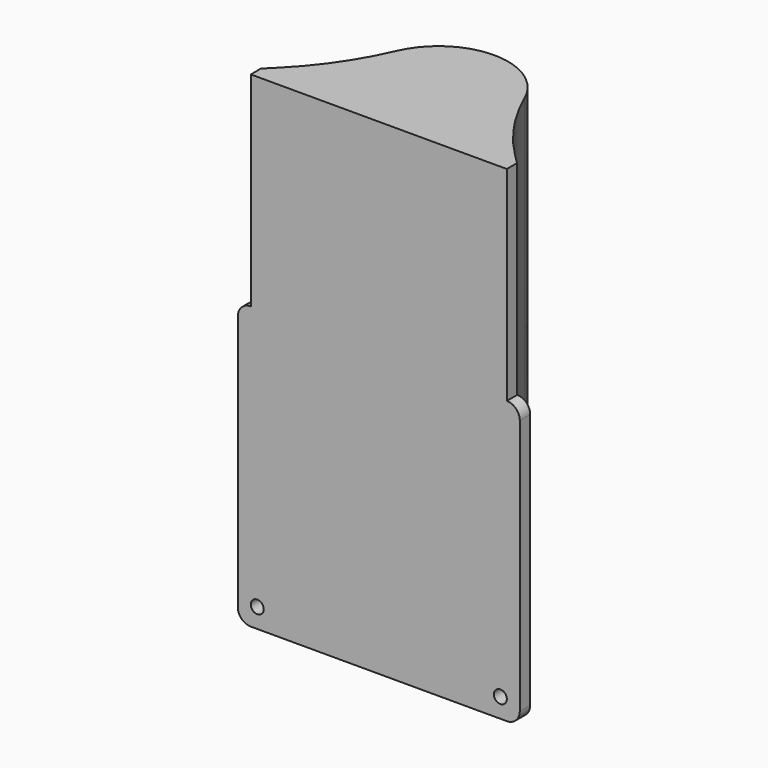
from build123d import *
from build123d import SkipClean  # not in build123d's __all__

# Parameters (mm, degrees)
F0_W           = 87
F0_H           = 87
F0_R           = 2
F1_DEPTH       = 4
F2_R           = 4
F5_DEPTH       = 43.5
F6_T1_DEPTH    = 87
F7_R           = 20.025
F8_DEPTH       = 87.001
F9_R           = 2
F10_DEPTH      = 40.501
F11_R          = 20
F12_DEPTH      = 10
F15_DEPTH      = 106.5
F15_DEPTH_BACK = 25.4
F16_R          = 20
F17_DEPTH      = 150.0010001
F18_R          = 20
F19_DEPTH      = 15


# Not quite as in the source:
# - a fillet or chamfer that OpenCascade refuses, or shapes differently, is made with other operations: its cross-section is extruded or revolved along the edge and cut away or added
# - after a boolean that leaves OpenCascade's solid faulty, fix() repairs it


with BuildPart() as f1:
    # F0 (on Front) → F1 (new body)
    with BuildSketch(Plane.XZ):
        Rectangle(F0_W, F0_H)
        with Locations((-37.5, -37.5)):
            Circle(F0_R, mode=Mode.SUBTRACT)
        with Locations((37.5, -37.5)):
            Circle(F0_R, mode=Mode.SUBTRACT)
        with Locations((-37.5, 37.5)):
            Circle(F0_R, mode=Mode.SUBTRACT)
        with Locations((37.5, 37.5)):
            Circle(F0_R, mode=Mode.SUBTRACT)
    extrude(amount=F1_DEPTH)

    # F2
    f2_edges = [f1.edges().sort_by_distance(p)[0] for p in [
        (43.5, -2, 43.5),
        (-43.5, -2, 43.5),
        (43.5, -2, -43.5),
        (-43.5, -2, -43.5),
    ]]
    fillet(f2_edges, radius=F2_R)

    # F4 (on Top) → F5 (join, symmetric)
    with BuildSketch(Plane.XY):
        with BuildLine():
            ThreePointArc((-10.0623058987, 0), (-17.7800410903, 6.9119836686), (-21.3690774705, 16.6309225295))
            Line((-21.3690774705, 16.6309225295), (-38, 0))
            Line((-38, 0), (-10.0623058987, 0))
        make_face()
        with BuildLine():
            Line((-38, 0), (-21.3690774705, 16.6309225295))
            ThreePointArc((-21.3690774705, 16.6309225295), (-21.4314768317, 17.2848321331), (-21.4738707868, 17.9403427756))
            Line((-21.4738707868, 17.9403427756), (-39.4142135624, 0))
            Line((-39.4142135624, 0), (-38, 0))
        make_face()
        with BuildLine():
            ThreePointArc((-21.4738707868, 17.9403427756), (-21.4314768317, 17.2848321331), (-21.3690774705, 16.6309225295))
            ThreePointArc((-21.3690774705, 16.6309225295), (-17.7800410903, 6.9119836686), (-10.0623058987, 0))
            Line((-10.0623058987, 0), (10.0623058987, 0))
            ThreePointArc((10.0623058987, 0), (17.7800410903, 6.9119836686), (21.3690774705, 16.6309225295))
            ThreePointArc((21.3690774705, 16.6309225295), (21.4314768317, 17.2848321331), (21.4738707868, 17.9403427756))
            Line((21.4738707868, 17.9403427756), (19.9956189847, 19.4185945777))
            ThreePointArc((19.9956189847, 19.4185945777), (13.9933575036, 33.2893647786), (0, 39))
            ThreePointArc((0, 39), (-13.9933575036, 33.2893647786), (-19.9956189847, 19.4185945777))
            Line((-19.9956189847, 19.4185945777), (-21.4738707868, 17.9403427756))
        make_face()
        with BuildLine():
            ThreePointArc((21.5, 19), (-0.5299896624, 40.493466704), (-21.4738707868, 17.9403427756))
            Line((-21.4738707868, 17.9403427756), (-19.9956189847, 19.4185945777))
            ThreePointArc((-19.9956189847, 19.4185945777), (-13.9933575036, 33.2893647786), (0, 39))
            ThreePointArc((0, 39), (13.9933575036, 33.2893647786), (19.9956189847, 19.4185945777))
            Line((19.9956189847, 19.4185945777), (21.4738707868, 17.9403427756))
            ThreePointArc((21.4738707868, 17.9403427756), (21.493466704, 18.4700103376), (21.5, 19))
        make_face()
        with BuildLine():
            Line((10.0623058987, 0), (-10.0623058987, 0))
            ThreePointArc((-10.0623058987, 0), (0, -2.5), (10.0623058987, 0))
        make_face()
        with BuildLine():
            ThreePointArc((21.3690774705, 16.6309225295), (17.7800410903, 6.9119836686), (10.0623058987, 0))
            Line((10.0623058987, 0), (38, 0))
            Line((38, 0), (21.3690774705, 16.6309225295))
        make_face()
        with BuildLine():
            Line((39.4142135624, 0), (21.4738707868, 17.9403427756))
            ThreePointArc((21.4738707868, 17.9403427756), (21.4314768317, 17.2848321331), (21.3690774705, 16.6309225295))
            Line((21.3690774705, 16.6309225295), (38, 0))
            Line((38, 0), (39.4142135624, 0))
        make_face()
    extrude(amount=F5_DEPTH, both=True)

    # F6: fillet of radius 80 on 2 edges, made by hand

    # F6_s2 → F6_t1 (join)
    with BuildSketch(Plane.XY.offset(-43.5)):
        with BuildLine():
            ThreePointArc((-36.5156161223, 2.89859744), (-26.9555540815, 14.444838104), (-19.7173340913, 27.5718572276))
            ThreePointArc((-19.7173340913, 27.5718572276), (-21.1511313524, 22.857413967), (-21.4738707868, 17.9403427756))
            Line((-21.4738707868, 17.9403427756), (-36.5156161223, 2.89859744))
        make_face()
        with BuildLine():
            ThreePointArc((19.7173340913, 27.5718572276), (26.9555540815, 14.444838104), (36.5156161223, 2.89859744))
            Line((36.5156161223, 2.89859744), (21.4738707868, 17.9403427756))
            ThreePointArc((21.4738707868, 17.9403427756), (21.1511313524, 22.857413967), (19.7173340913, 27.5718572276))
        make_face()
    extrude(amount=F6_T1_DEPTH)

    # F7 (on face) → F8 (cut, through all)
    with BuildSketch(Plane.XY.offset(43.5)):
        with Locations((0, 19)):
            Circle(F7_R)
    extrude(amount=-F8_DEPTH, mode=Mode.SUBTRACT)

    # F9 (on Front) → F10 (cut, through all)
    with BuildSketch(Plane.XZ):
        with BuildLine():
            Line((-37.5, 35.5), (-37.5, 37.5))
            Line((-37.5, 37.5), (-35.5, 37.5))
            ThreePointArc((-35.5, 37.5), (-38.9142135624, 38.9142135624), (-37.5, 35.5))
        make_face()
        with BuildLine():
            Line((-35.5, 37.5), (-37.5, 37.5))
            Line((-37.5, 37.5), (-37.5, 35.5))
            ThreePointArc((-37.5, 35.5), (-36.0857864376, 36.0857864376), (-35.5, 37.5))
        make_face()
        with BuildLine():
            ThreePointArc((39.5, 37.5), (37.5, 39.5), (35.5, 37.5))
            ThreePointArc((35.5, 37.5), (37.5, 35.5), (39.5, 37.5))
        make_face()
        with BuildLine():
            ThreePointArc((-35.5, -37.5), (-36.0857864376, -36.0857864376), (-37.5, -35.5))
            ThreePointArc((-37.5, -35.5), (-38.9142135624, -38.9142135624), (-35.5, -37.5))
        make_face()
        with Locations((37.5, -37.5)):
            Circle(F9_R)
    with SkipClean():  # cleaning this boolean's faces spoils the solid; the shape is the same uncleaned
        extrude(amount=-F10_DEPTH, mode=Mode.SUBTRACT)

    # F14 (on Top) → F15 (join, two sides)
    with BuildSketch(Plane.XY) as f15_sk:
        with BuildLine():
            Line((-39.5, -4), (39.5, -4))
            Line((39.5, -4), (39.5, 0))
            Line((39.5, 0), (39.4142135624, 0))
            Line((39.4142135624, 0), (36.5156161223, 2.89859744))
            ThreePointArc((36.5156161223, 2.89859744), (26.9555540815, 14.444838104), (19.7173340913, 27.5718572276))
            ThreePointArc((19.7173340913, 27.5718572276), (0, 40.5), (-19.7173340913, 27.5718572276))
            ThreePointArc((-19.7173340913, 27.5718572276), (-26.9555540815, 14.444838104), (-36.5156161223, 2.89859744))
            Line((-36.5156161223, 2.89859744), (-39.4142135624, 0))
            Line((-39.4142135624, 0), (-39.5, 0))
            Line((-39.5, 0), (-39.5, -4))
        make_face()
    extrude(amount=F15_DEPTH)
    extrude(f15_sk.sketch, amount=-F15_DEPTH_BACK)

    add(f1.part.fix(), mode=Mode.REPLACE)

    # F16 (on face) → F17 (cut, through all)
    with BuildSketch(Plane.XY.offset(106.5)):
        with Locations((0, 19)):
            Circle(F16_R)
    extrude(amount=-F17_DEPTH, mode=Mode.SUBTRACT)

    # F18 (on face) → F19 (join)
    with BuildSketch(Plane.XY.offset(106.5)):
        with Locations((0, 19)):
            Circle(F18_R)
    extrude(amount=-F19_DEPTH)


with BuildPart() as f12:
    # F11 (on face) → F12 (new body)
    with BuildSketch(Plane(origin=(0, 0, -43.5), x_dir=(1, 0, 0), z_dir=(0, 0, -1))):
        with Locations((0, -19)):
            Circle(F11_R)
    extrude(amount=-F12_DEPTH)


solid = f1.part
